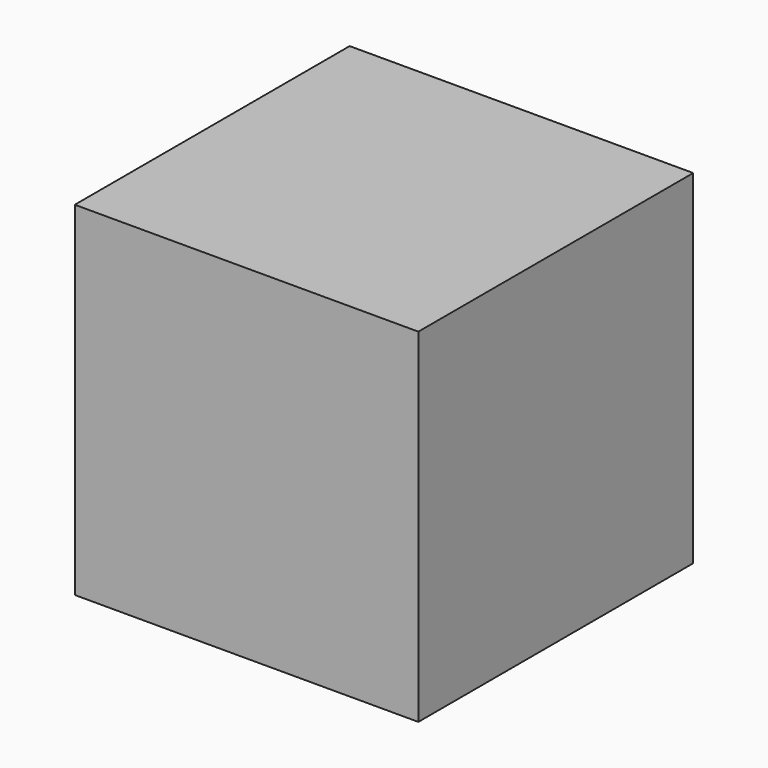
from build123d import *

# Parameters (mm, degrees)
F1_W     = 5
F1_H     = 5
F2_DEPTH = 5


with BuildPart() as f2:
    # F1 (on Front) → F2 (new body)
    with BuildSketch(Plane.XZ):
        with Locations((0.075369142, -0.1677119303)):
            Rectangle(F1_W, F1_H)
    extrude(amount=F2_DEPTH)


solid = f2.part
